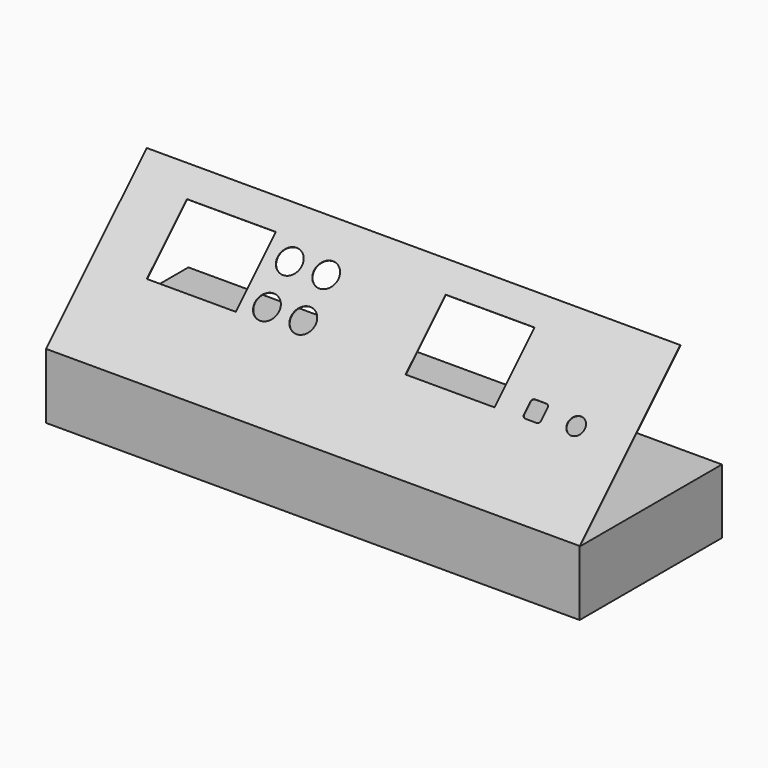
from build123d import *

# Parameters (mm, degrees)
F1_DEPTH = 209.55
F2_W     = 69.85
F2_H     = 55.5625
F3_DEPTH = 0.4064


# Not quite as in the source:
# - the dataset's text gives a spline's control points without its knots; the knots are read off the source's solid


with BuildPart() as f1:
    # F0 (on Right) → F1 (new body, symmetric)
    with BuildSketch(Plane.YZ):
        Polygon((-139.7, 0), (0, 0), (0, 50.8), (-139.2936, 50.8), (-139.2936, 51.054), (-40.6298144724, 149.7177855276), (-40.9171826682, 150.0051537235), (-139.7, 51.2223363917), align=None)
    extrude(amount=F1_DEPTH, both=True)

    # F2 (on face) → F3 (cut, through all)
    with BuildSketch(Plane(origin=(0, -95.4611681959, 95.4611681959), x_dir=(1, 0, 0), z_dir=(0, -0.7071067812, 0.7071067812))):
        with Locations((-131.0096597559, 28.0834854854)):
            Rectangle(F2_W, F2_H)
        Polygon((107.1301484441, 55.8647354854), (37.2801484441, 55.8647354854), (37.2801484441, 0.3022354854), (107.1301484441, 0.3022354854), (107.1301484441, 6.5523372854), (107.1301484441, 32.9500238854), align=None)
        with BuildLine():
            add(Edge.make_bspline(
                [(129.6562400441, 13.0987046854), (129.2159818441, 12.6577352854), (128.9582734441, 12.0382800854), (128.9582734441, 11.4147354854)],
                knots=[1, 1, 1, 1, 2, 2, 2, 2], degree=3))
            Line((128.9582734441, 11.4147354854), (128.9582734441, 2.6834854854))
            add(Edge.make_bspline(
                [(128.9582734441, 2.6834854854), (128.9582734441, 2.0599154854), (129.2159818441, 1.4404856854), (129.6562400441, 1.0002274854)],
                knots=[0, 0, 0, 0, 1, 1, 1, 1], degree=3))
            add(Edge.make_bspline(
                [(129.6562400441, 1.0002274854), (130.0972094441, 0.5592326854), (130.7166646441, 0.3022354854), (131.3395234441, 0.3022354854)],
                knots=[1, 1, 1, 1, 2, 2, 2, 2], degree=3))
            Line((131.3395234441, 0.3022354854), (140.0707734441, 0.3022354854))
            add(Edge.make_bspline(
                [(140.0707734441, 0.3022354854), (140.6950038441, 0.3022354854), (141.3137478441, 0.5592326854), (141.7547172441, 1.0002274854)],
                knots=[0, 0, 0, 0, 1, 1, 1, 1], degree=3))
            add(Edge.make_bspline(
                [(141.7547172441, 1.0002274854), (142.1956866441, 1.4404856854), (142.4520234441, 2.0599154854), (142.4520234441, 2.6834854854)],
                knots=[1, 1, 1, 1, 2, 2, 2, 2], degree=3))
            Line((142.4520234441, 2.6834854854), (142.4520234441, 11.4147354854))
            add(Edge.make_bspline(
                [(142.4520234441, 11.4147354854), (142.4520234441, 12.0382800854), (142.1956866441, 12.6577352854), (141.7547172441, 13.0987046854), (141.3137478441, 13.5396740854), (140.6950038441, 13.7959854854), (140.0707734441, 13.7959854854)],
                knots=[0, 0, 0, 0, 1, 1, 1, 2, 2, 2, 2], degree=3))
            Line((140.0707734441, 13.7959854854), (131.3395234441, 13.7959854854))
            add(Edge.make_bspline(
                [(131.3395234441, 13.7959854854), (130.7166646441, 13.7959854854), (130.0972094441, 13.5396740854), (129.6562400441, 13.0987046854)],
                knots=[0, 0, 0, 0, 1, 1, 1, 1], degree=3))
        make_face()
        with BuildLine():
            add(Edge.make_bspline(
                [(-70.2991639559, 48.3124010854), (-72.0623811559, 50.0755928854), (-74.5410909559, 51.1022354854), (-77.0346597559, 51.1022354854)],
                knots=[7, 7, 7, 7, 8, 8, 8, 8], degree=3))
            add(Edge.make_bspline(
                [(-77.0346597559, 51.1022354854), (-79.5278983559, 51.1022354854), (-82.0066589559, 50.0755928854), (-83.7698253559, 48.3124010854), (-85.5330171559, 46.5491838854), (-86.5596597559, 44.0707788854), (-86.5596597559, 41.5772354854), (-86.5596597559, 39.0836666854), (-85.5330171559, 36.6052616854), (-83.7698253559, 34.8420952854)],
                knots=[0, 0, 0, 0, 1, 1, 1, 2, 2, 2, 3, 3, 3, 3], degree=3))
            add(Edge.make_bspline(
                [(-83.7698253559, 34.8420952854), (-82.0066589559, 33.0788526854), (-79.5278983559, 32.0522354854), (-77.0346597559, 32.0522354854), (-74.5410909559, 32.0522354854), (-72.0623811559, 33.0788526854), (-70.2991639559, 34.8420952854)],
                knots=[3, 3, 3, 3, 4, 4, 4, 5, 5, 5, 5], degree=3))
            add(Edge.make_bspline(
                [(-70.2991639559, 34.8420952854), (-68.5359721559, 36.6052616854), (-67.5096597559, 39.0836666854), (-67.5096597559, 41.5772354854), (-67.5096597559, 44.0707788854), (-68.5359721559, 46.5491838854), (-70.2991639559, 48.3124010854)],
                knots=[5, 5, 5, 5, 6, 6, 6, 7, 7, 7, 7], degree=3))
        make_face()
        with BuildLine():
            add(Edge.make_bspline(
                [(-70.2991639559, 16.5624010854), (-72.0623811559, 18.3255928854), (-74.5410909559, 19.3522354854), (-77.0346597559, 19.3522354854)],
                knots=[7, 7, 7, 7, 8, 8, 8, 8], degree=3))
            add(Edge.make_bspline(
                [(-77.0346597559, 19.3522354854), (-79.5278983559, 19.3522354854), (-82.0066589559, 18.3255928854), (-83.7698253559, 16.5624010854), (-85.5330171559, 14.7991838854), (-86.5596597559, 12.3207788854), (-86.5596597559, 9.8272354854), (-86.5596597559, 7.3336666854), (-85.5330171559, 4.8552616854), (-83.7698253559, 3.0920952854)],
                knots=[0, 0, 0, 0, 1, 1, 1, 2, 2, 2, 3, 3, 3, 3], degree=3))
            add(Edge.make_bspline(
                [(-83.7698253559, 3.0920952854), (-82.0066589559, 1.3288526854), (-79.5278983559, 0.3022354854), (-77.0346597559, 0.3022354854), (-74.5410909559, 0.3022354854), (-72.0623811559, 1.3288526854), (-70.2991639559, 3.0920952854)],
                knots=[3, 3, 3, 3, 4, 4, 4, 5, 5, 5, 5], degree=3))
            add(Edge.make_bspline(
                [(-70.2991639559, 3.0920952854), (-68.5359721559, 4.8552616854), (-67.5096597559, 7.3336666854), (-67.5096597559, 9.8272354854), (-67.5096597559, 12.3207788854), (-68.5359721559, 14.7991838854), (-70.2991639559, 16.5624010854)],
                knots=[5, 5, 5, 5, 6, 6, 6, 7, 7, 7, 7], degree=3))
        make_face()
        with BuildLine():
            add(Edge.make_bspline(
                [(-41.7090255559, 16.5624010854), (-43.4721919559, 18.3255928854), (-45.9506223559, 19.3522354854), (-48.4441911559, 19.3522354854)],
                knots=[7, 7, 7, 7, 8, 8, 8, 8], degree=3))
            add(Edge.make_bspline(
                [(-48.4441911559, 19.3522354854), (-50.9380647559, 19.3522354854), (-53.4164697559, 18.3255928854), (-55.1796615559, 16.5624010854), (-56.9428787559, 14.7991838854), (-57.9691911559, 12.3207788854), (-57.9691911559, 9.8272354854), (-57.9691911559, 7.3336666854), (-56.9428787559, 4.8552616854), (-55.1796615559, 3.0920952854)],
                knots=[0, 0, 0, 0, 1, 1, 1, 2, 2, 2, 3, 3, 3, 3], degree=3))
            add(Edge.make_bspline(
                [(-55.1796615559, 3.0920952854), (-53.4164697559, 1.3288526854), (-50.9380647559, 0.3022354854), (-48.4441911559, 0.3022354854), (-45.9506223559, 0.3022354854), (-43.4721919559, 1.3288526854), (-41.7090255559, 3.0920952854)],
                knots=[3, 3, 3, 3, 4, 4, 4, 5, 5, 5, 5], degree=3))
            add(Edge.make_bspline(
                [(-41.7090255559, 3.0920952854), (-39.9454527559, 4.8552616854), (-38.9194959559, 7.3336666854), (-38.9194959559, 9.8272354854), (-38.9194959559, 12.3207788854), (-39.9454527559, 14.7991838854), (-41.7090255559, 16.5624010854)],
                knots=[5, 5, 5, 5, 6, 6, 6, 7, 7, 7, 7], degree=3))
        make_face()
        with BuildLine():
            add(Edge.make_bspline(
                [(-41.7090255559, 48.3124010854), (-43.4721919559, 50.0755928854), (-45.9506223559, 51.1022354854), (-48.4441911559, 51.1022354854)],
                knots=[7, 7, 7, 7, 8, 8, 8, 8], degree=3))
            add(Edge.make_bspline(
                [(-48.4441911559, 51.1022354854), (-50.9380647559, 51.1022354854), (-53.4164697559, 50.0755928854), (-55.1796615559, 48.3124010854), (-56.9428787559, 46.5491838854), (-57.9691911559, 44.0707788854), (-57.9691911559, 41.5772354854), (-57.9691911559, 39.0836666854), (-56.9428787559, 36.6052616854), (-55.1796615559, 34.8420952854)],
                knots=[0, 0, 0, 0, 1, 1, 1, 2, 2, 2, 3, 3, 3, 3], degree=3))
            add(Edge.make_bspline(
                [(-55.1796615559, 34.8420952854), (-53.4164697559, 33.0788526854), (-50.9380647559, 32.0522354854), (-48.4441911559, 32.0522354854), (-45.9506223559, 32.0522354854), (-43.4721919559, 33.0788526854), (-41.7090255559, 34.8420952854)],
                knots=[3, 3, 3, 3, 4, 4, 4, 5, 5, 5, 5], degree=3))
            add(Edge.make_bspline(
                [(-41.7090255559, 34.8420952854), (-39.9454527559, 36.6052616854), (-38.9194959559, 39.0836666854), (-38.9194959559, 41.5772354854), (-38.9194959559, 44.0707788854), (-39.9454527559, 46.5491838854), (-41.7090255559, 48.3124010854)],
                knots=[5, 5, 5, 5, 6, 6, 6, 7, 7, 7, 7], degree=3))
        make_face()
        with BuildLine():
            add(Edge.make_bspline(
                [(172.2259034441, 11.8198654854), (170.9774172441, 13.0690628854), (169.2224804441, 13.7959854854), (167.4551484441, 13.7959854854)],
                knots=[7, 7, 7, 7, 8, 8, 8, 8], degree=3))
            add(Edge.make_bspline(
                [(167.4551484441, 13.7959854854), (165.6891880441, 13.7959854854), (163.9342512441, 13.0690628854), (162.6850538441, 11.8198654854)],
                knots=[0, 0, 0, 0, 1, 1, 1, 1], degree=3))
            add(Edge.make_bspline(
                [(162.6850538441, 11.8198654854), (161.4358818441, 10.5713538854), (160.7082734441, 8.8157566854), (160.7082734441, 7.0491104854), (160.7082734441, 5.2831500854), (161.4358818441, 3.5275274854), (162.6850538441, 2.2783300854)],
                knots=[1, 1, 1, 1, 2, 2, 2, 3, 3, 3, 3], degree=3))
            add(Edge.make_bspline(
                [(162.6850538441, 2.2783300854), (163.9342512441, 1.0298438854), (165.6891880441, 0.3022354854), (167.4551484441, 0.3022354854), (169.2224804441, 0.3022354854), (170.9774172441, 1.0298438854), (172.2259034441, 2.2783300854)],
                knots=[3, 3, 3, 3, 4, 4, 4, 5, 5, 5, 5], degree=3))
            add(Edge.make_bspline(
                [(172.2259034441, 2.2783300854), (173.4750754441, 3.5275274854), (174.2020234441, 5.2831500854), (174.2020234441, 7.0491104854), (174.2020234441, 8.8157566854), (173.4750754441, 10.5713538854), (172.2259034441, 11.8198654854)],
                knots=[5, 5, 5, 5, 6, 6, 6, 7, 7, 7, 7], degree=3))
        make_face()
    extrude(amount=-F3_DEPTH, mode=Mode.SUBTRACT)


solid = f1.part
